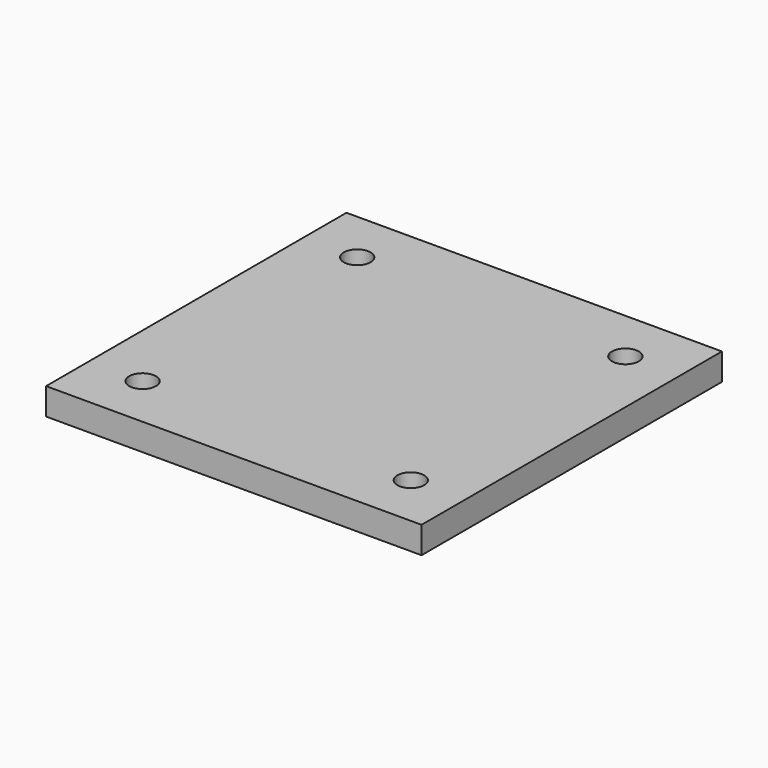
from build123d import *

# Parameters (mm, degrees)
F0_W     = 355.6
F0_H     = 355.6
F1_DEPTH = 25.4
F4_D     = 25.4


# Not quite as in the source:
# - the program builds the solid bodies; features that only make, move or delete a surface that nothing else refers to are left out


with BuildPart() as f1:
    # F0 (on Top) → F1 (new body)
    with BuildSketch(Plane.XY):
        Rectangle(F0_W, F0_H)
    extrude(amount=F1_DEPTH)

    # F4 (through all)
    with Locations(Plane.XY.offset(25.4)):
        with Locations((-127, -127), (127, -127), (127, 127), (-127, 127)):
            Hole(F4_D / 2)


solid = f1.part
